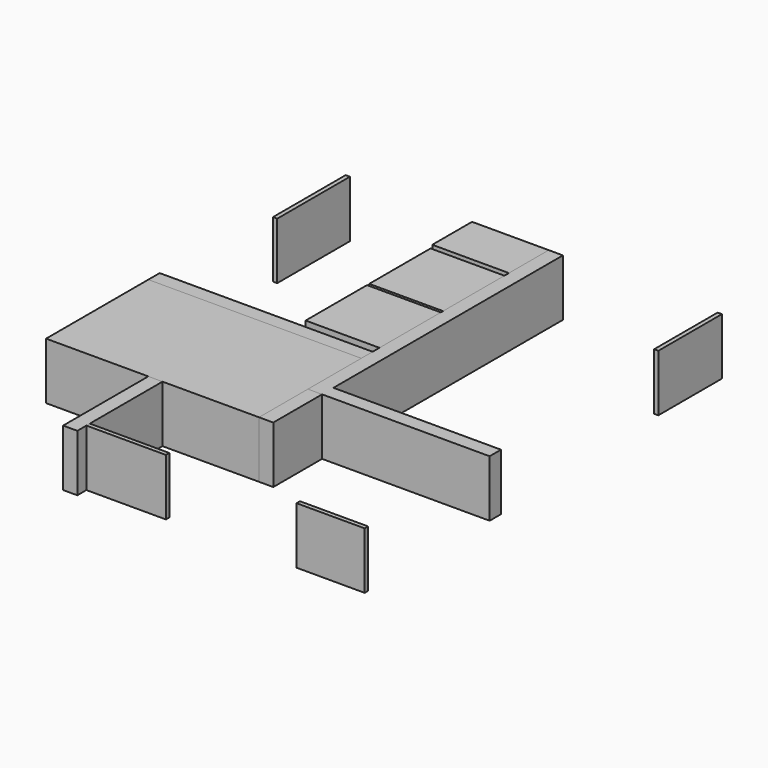
from build123d import *

# Parameters (mm, degrees)
F9_W      = 1905
F9_H      = 1143
F12_DEPTH = 508
F8_W      = 1905
F8_H      = 127
F7_W      = 127
F7_H      = 952.5
F4_W      = 660.4
F4_H      = 685.8
F1_W      = 685.8
F1_H      = 444.5
F10_W     = 127
F10_H     = 546.1
F2_W      = 127
F2_H      = 2565.4
F13_DEPTH = 508


# Not quite as in the source:
# - the program builds the solid bodies; features that only make, move or delete a surface that nothing else refers to are left out


with BuildPart() as f12:
    # F9 (on face) → F12 (new body)
    with BuildSketch(Plane.XY):
        with Locations((-831.9651317239, -767.9497311732)):
            Rectangle(F9_W, F9_H)
    extrude(amount=F12_DEPTH)


with BuildPart() as f12b:
    # F8 (on Top) → F12, piece 2 (new body)
    with BuildSketch(Plane.XY):
        with Locations((-831.9651317239, -132.9497311732)):
            Rectangle(F8_W, F8_H)
    extrude(amount=F12_DEPTH)


with BuildPart() as f12c:
    # F7 (on Top) → F12, piece 3 (new body)
    with BuildSketch(Plane.XY):
        with Locations((-806.5651317239, -1815.6997311732)):
            Rectangle(F7_W, F7_H)
    extrude(amount=F12_DEPTH)


with BuildPart() as f12d:
    # F6 (on Top) → F12, piece 4 (new body)
    with BuildSketch(Plane.XY):
        with BuildLine():
            Line((-1657.4651317239, 1899.0502688268), (-1695.5651317239, 1899.0502688268))
            Line((-1695.5651317239, 1899.0502688268), (-1695.5651317239, 1086.2502688268))
            ThreePointArc((-1695.5651317239, 1086.2502688268), (-1676.5098944488, 1086.4736644797), (-1657.4651317239, 1087.1437286389))
            Line((-1657.4651317239, 1087.1437286389), (-1657.4651317239, 1899.0502688268))
        make_face()
        with BuildLine():
            ThreePointArc((-1657.4651317239, 1087.1437286389), (-1676.5098944488, 1086.4736644797), (-1695.5651317239, 1086.2502688268))
            Line((-1695.5651317239, 1086.2502688268), (-1657.4651317239, 1086.2502688268))
            Line((-1657.4651317239, 1086.2502688268), (-1657.4651317239, 1087.1437286389))
        make_face()
    extrude(amount=F12_DEPTH)


with BuildPart() as f12e:
    # F5 (on Top) → F12, piece 5 (new body)
    with BuildSketch(Plane.XY):
        with BuildLine():
            Line((1669.9348682761, 1187.8502688268), (1669.9348682761, 1899.0502688268))
            Line((1669.9348682761, 1899.0502688268), (1631.8348682761, 1899.0502688268))
            Line((1631.8348682761, 1899.0502688268), (1631.8348682761, 1188.871537802))
            ThreePointArc((1631.8348682761, 1188.871537802), (1650.8780257365, 1188.1056319159), (1669.9348682761, 1187.8502688268))
        make_face()
        with BuildLine():
            Line((1631.8348682761, 1187.8502688268), (1669.9348682761, 1187.8502688268))
            ThreePointArc((1669.9348682761, 1187.8502688268), (1650.8780257365, 1188.1056319159), (1631.8348682761, 1188.871537802))
            Line((1631.8348682761, 1188.871537802), (1631.8348682761, 1187.8502688268))
        make_face()
    extrude(amount=F12_DEPTH)


with BuildPart() as f12f:
    # F4 (on Top) → F12, piece 6 (new body)
    with BuildSketch(Plane.XY):
        with Locations((-209.6651317239, 349.6502688268)):
            Rectangle(F4_W, F4_H)
    extrude(amount=F12_DEPTH)


with BuildPart() as f12g:
    # F4 (on Top) → F12, piece 7 (new body)
    with BuildSketch(Plane.XY):
        with Locations((-209.6651317239, 1060.8502688268)):
            Rectangle(F4_W, F4_H)
    extrude(amount=F12_DEPTH)


with BuildPart() as f12h:
    # F3 (on Top) → F12, piece 8 (new body)
    with BuildSketch(Plane.XY):
        with BuildLine():
            Line((1137.7266582723, -2152.2497311732), (1136.5348682761, -2152.2497311732))
            Line((1136.5348682761, -2152.2497311732), (1136.5348682761, -2190.3497311732))
            ThreePointArc((1136.5348682761, -2190.3497311732), (1136.832888623, -2171.2904134821), (1137.7266582723, -2152.2497311732))
        make_face()
        with BuildLine():
            Line((1746.1348682761, -2152.2497311732), (1137.7266582723, -2152.2497311732))
            ThreePointArc((1137.7266582723, -2152.2497311732), (1136.832888623, -2171.2904134821), (1136.5348682761, -2190.3497311732))
            Line((1136.5348682761, -2190.3497311732), (1746.1348682761, -2190.3497311732))
            Line((1746.1348682761, -2190.3497311732), (1746.1348682761, -2152.2497311732))
        make_face()
    extrude(amount=F12_DEPTH)


with BuildPart() as f12i:
    # F1 (on Top) → F12, piece 9 (new body)
    with BuildSketch(Plane.XY):
        with Locations((-222.3651317239, 1676.8002688268)):
            Rectangle(F1_W, F1_H)
    extrude(amount=F12_DEPTH)


with BuildPart() as f12j:
    # F10 (on face) → F12, piece 10 (new body)
    with BuildSketch(Plane.XY):
        with Locations((184.0348682761, -1066.3997311732)):
            Rectangle(F10_W, F10_H)
    extrude(amount=F12_DEPTH)


with BuildPart() as f12k:
    # F11 (on face) → F12, piece 11 (new body)
    with BuildSketch(Plane.XY):
        with BuildLine():
            Line((-743.0651317239, -2152.2497311732), (-743.0651317239, -2190.3497311732))
            Line((-743.0651317239, -2190.3497311732), (-31.8651317239, -2190.3497311732))
            ThreePointArc((-31.8651317239, -2190.3497311732), (-32.1204948129, -2171.2928886335), (-32.8864006991, -2152.2497311732))
            Line((-32.8864006991, -2152.2497311732), (-743.0651317239, -2152.2497311732))
        make_face()
        with BuildLine():
            ThreePointArc((-32.8864006991, -2152.2497311732), (-32.1204948129, -2171.2928886335), (-31.8651317239, -2190.3497311732))
            Line((-31.8651317239, -2190.3497311732), (-31.8651317239, -2152.2497311732))
            Line((-31.8651317239, -2152.2497311732), (-32.8864006991, -2152.2497311732))
        make_face()
    extrude(amount=F12_DEPTH)


with BuildPart() as f13:
    # F2 (on Top) → F13 (new body)
    with BuildSketch(Plane.XY):
        with Locations((184.0348682761, 616.3502688268)):
            Rectangle(F2_W, F2_H)
        Polygon((247.5348682761, -793.3497311732), (1746.1348682761, -793.3497311732), (1746.1348682761, -666.3497311732), (247.5348682761, -666.3497311732), (120.5348682761, -666.3497311732), (120.5348682761, -793.3497311732), align=None)
    extrude(amount=F13_DEPTH)


solid = Compound([f12.part, f12b.part, f12c.part, f12d.part, f12e.part, f12f.part, f12g.part, f12h.part, f12i.part, f12j.part, f12k.part, f13.part])
